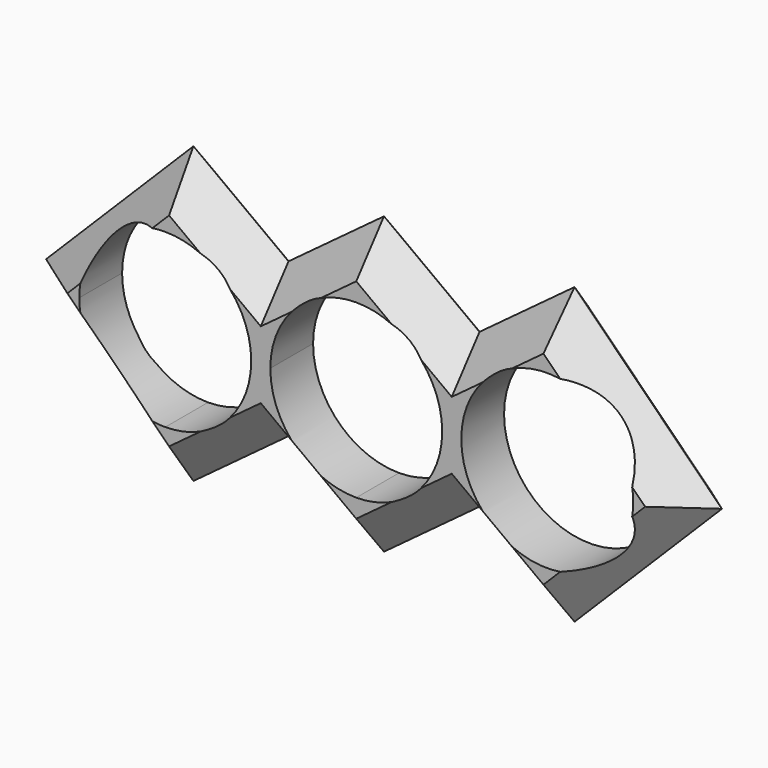
from build123d import *

# Parameters (mm, degrees)
F1_DEPTH      = 7
F2_T1_DEPTH   = 54.4125704052
F2_T3_DEPTH   = 54.4125704052
F2_T5_DEPTH   = 54.4125704052
F2_T7_DEPTH   = 54.4125704052
F2_T12_DEPTH  = 41.6814695772
F2_T17_DEPTH  = 41.6814695772
F2_T22_DEPTH  = 41.6814695772
F2_T27_DEPTH  = 41.6814695772
F2_T32_DEPTH  = 41.6814695772
F2_T37_DEPTH  = 41.6814695772
F2_T42_DEPTH  = 41.6814695772
F2_T47_DEPTH  = 41.6814695772
F2_T53_DEPTH  = 41.6814695772
F2_S55_R      = 11.25
F2_T56_DEPTH  = 25
F2_T59_DEPTH  = 41.6814695772
F2_S61_R      = 11.25
F2_T62_DEPTH  = 25
F2_T68_DEPTH  = 41.6814695772
F2_S70_R      = 11.25
F2_T71_DEPTH  = 25
F2_T74_DEPTH  = 41.6814695772
F2_S76_R      = 11.25
F2_T77_DEPTH  = 25
F2_T83_DEPTH  = 41.6814695772
F2_S85_R      = 11.25
F2_T86_DEPTH  = 25
F2_T89_DEPTH  = 41.6814695772
F2_S91_R      = 11.25
F2_T92_DEPTH  = 25
F2_T98_DEPTH  = 41.6814695772
F2_S100_R     = 11.25
F2_T101_DEPTH = 25
F2_T104_DEPTH = 41.6814695772
F2_S106_R     = 11.25
F2_T107_DEPTH = 25
F3_T1_DEPTH   = 43.7143691753
F3_T3_DEPTH   = 43.7143691753
F3_T5_DEPTH   = 43.7143691753
F3_T7_DEPTH   = 43.7143691753
F3_T12_DEPTH  = 30.9832683473
F3_T17_DEPTH  = 30.9832683473
F3_T22_DEPTH  = 30.9832683473
F3_T27_DEPTH  = 30.9832683473
F3_T32_DEPTH  = 30.9832683473
F3_T37_DEPTH  = 30.9832683473
F3_T42_DEPTH  = 30.9832683473
F3_T47_DEPTH  = 30.9832683473
F3_T53_DEPTH  = 30.9832683473
F3_T57_DEPTH  = 30.9832683473
F3_T64_DEPTH  = 30.9832683473
F3_T68_DEPTH  = 30.9832683473
F3_T75_DEPTH  = 30.9832683473
F3_T79_DEPTH  = 30.9832683473
F3_T86_DEPTH  = 30.9832683473
F3_T90_DEPTH  = 30.9832683473


# Not quite as in the source:
# - a fillet or chamfer that OpenCascade refuses, or shapes differently, is made with other operations: its cross-section is extruded or revolved along the edge and cut away or added


with BuildPart() as f1:
    # F0 (on Front) → F1 (new body)
    with BuildSketch(Plane.XZ):
        with BuildLine():
            Line((-25, 11.25), (-25, 20))
            Line((-25, 20), (-45, 0))
            Line((-45, 0), (-36.25, 0))
            ThreePointArc((-36.25, 0), (-32.9549512883, 7.9549512883), (-25, 11.25))
        make_face()
        with BuildLine():
            Line((-13.75, 0), (-12.5, 0))
            Line((-12.5, 0), (-12.5, 10.7452115044))
            Line((-12.5, 10.7452115044), (-25, 20))
            Line((-25, 20), (-25, 11.25))
            ThreePointArc((-25, 11.25), (-17.0450487117, 7.9549512883), (-13.75, 0))
        make_face()
        with BuildLine():
            Line((-12.5, -10.7452115044), (-12.5, 0))
            Line((-12.5, 0), (-13.75, 0))
            ThreePointArc((-13.75, 0), (-17.0450487117, -7.9549512883), (-25, -11.25))
            Line((-25, -11.25), (-25, -20))
            Line((-25, -20), (-12.5, -10.7452115044))
        make_face()
        with BuildLine():
            Line((-45, 0), (-25, -20))
            Line((-25, -20), (-25, -11.25))
            ThreePointArc((-25, -11.25), (-32.9549512883, -7.9549512883), (-36.25, 0))
            Line((-36.25, 0), (-45, 0))
        make_face()
        with BuildLine():
            Line((0, -20), (0, -11.25))
            ThreePointArc((0, -11.25), (-7.9549512883, -7.9549512883), (-11.25, 0))
            Line((-11.25, 0), (-12.5, 0))
            Line((-12.5, 0), (-12.5, -10.7452115044))
            Line((-12.5, -10.7452115044), (0, -20))
        make_face()
        with BuildLine():
            Line((12.5, 0), (11.25, 0))
            ThreePointArc((11.25, 0), (7.9549512883, -7.9549512883), (0, -11.25))
            Line((0, -11.25), (0, -20))
            Line((0, -20), (12.5, -10.7452115044))
            Line((12.5, -10.7452115044), (12.5, 0))
        make_face()
        with BuildLine():
            ThreePointArc((0, 11.25), (7.9549512883, 7.9549512883), (11.25, 0))
            Line((11.25, 0), (12.5, 0))
            Line((12.5, 0), (12.5, 10.7452115044))
            Line((12.5, 10.7452115044), (0, 20))
            Line((0, 20), (0, 11.25))
        make_face()
        with BuildLine():
            ThreePointArc((-11.25, 0), (-7.9549512883, 7.9549512883), (0, 11.25))
            Line((0, 11.25), (0, 20))
            Line((0, 20), (-12.5, 10.7452115044))
            Line((-12.5, 10.7452115044), (-12.5, 0))
            Line((-12.5, 0), (-11.25, 0))
        make_face()
        with BuildLine():
            Line((12.5, 10.7452115044), (12.5, 0))
            Line((12.5, 0), (13.75, 0))
            ThreePointArc((13.75, 0), (25, 11.25), (36.25, 0))
            Line((36.25, 0), (45, 0))
            Line((45, 0), (25, 20))
            Line((25, 20), (12.5, 10.7452115044))
        make_face()
        with BuildLine():
            Line((13.75, 0), (12.5, 0))
            Line((12.5, 0), (12.5, -10.7452115044))
            Line((12.5, -10.7452115044), (25, -20))
            Line((25, -20), (45, 0))
            Line((45, 0), (36.25, 0))
            ThreePointArc((36.25, 0), (25, -11.25), (13.75, 0))
        make_face()
    extrude(amount=F1_DEPTH)

    # F2: chamfer of 5.08 on 12 edges, made by hand

    # F2_s2 → F2_t1 (cut)
    with BuildSketch(Plane(origin=(6.7377487577, 0, 6.7377487577), x_dir=(0, 1, 0), z_dir=(-0.7071067812, 0, -0.7071067812))):
        Polygon((-1.92, -31.8198051534), (-7, -26.7398051534), (-7, -31.8198051534), align=None)
    extrude(amount=F2_T1_DEPTH, mode=Mode.SUBTRACT)

    # F2_s4 → F2_t3 (cut)
    with BuildSketch(Plane(origin=(31.7377487577, 0, -31.7377487577), x_dir=(0, 1, 0), z_dir=(-0.7071067812, 0, 0.7071067812))):
        Polygon((-1.92, -31.8198051534), (-7, -26.7398051534), (-7, -31.8198051534), align=None)
    extrude(amount=F2_T3_DEPTH, mode=Mode.SUBTRACT)

    # F2_s6 → F2_t5 (cut)
    with BuildSketch(Plane(origin=(-6.7377487577, 0, -6.7377487577), x_dir=(0, 1, 0), z_dir=(0.7071067812, 0, 0.7071067812))):
        Polygon((-1.92, -31.8198051534), (-7, -26.7398051534), (-7, -31.8198051534), align=None)
    extrude(amount=F2_T5_DEPTH, mode=Mode.SUBTRACT)

    # F2_s8 → F2_t7 (cut)
    with BuildSketch(Plane(origin=(-31.7377487577, 0, 31.7377487577), x_dir=(0, 1, 0), z_dir=(0.7071067812, 0, -0.7071067812))):
        Polygon((-1.92, -31.8198051534), (-7, -26.7398051534), (-7, -31.8198051534), align=None)
    extrude(amount=F2_T7_DEPTH, mode=Mode.SUBTRACT)


with BuildPart() as f2_tool10:
    # F2_s11 → F2_t12 (new body)
    with BuildSketch(Plane(origin=(-2.7131807604, 0, 2.008793127), x_dir=(0, 1, 0), z_dir=(-0.8036946592, 0, 0.5950419269))):
        Polygon((-1.92, -1.1978450121), (-7, 3.8821549879), (-7, -1.1978450121), align=None)
    extrude(amount=F2_T12_DEPTH)

    split(bisect_by=Plane(origin=(-9.5646403729, 0, 12.918502105), x_dir=(0, 1, 0), z_dir=(-0.5950419269, 0, 0.8036946592)), keep=Keep.TOP)


with BuildPart() as f1_1:
    add(f1.part)

    # F2_t9: cut F2_tool10
    add(f2_tool10.part, mode=Mode.SUBTRACT)


with BuildPart() as f2_tool15:
    # F2_s16 → F2_t17 (new body)
    with BuildSketch(Plane(origin=(20.0642276166, 0, 14.8552146336), x_dir=(0, 1, 0), z_dir=(-0.8036946592, 0, -0.5950419269))):
        Polygon((-1.92, -16.0738931843), (-7, -10.9938931843), (-7, -16.0738931843), align=None)
    extrude(amount=F2_T17_DEPTH)

    split(bisect_by=Plane(origin=(0.7127680041, 0, 0.9627016388), x_dir=(0, 1, 0), z_dir=(0.5950419269, 0, 0.8036946592)), keep=Keep.TOP)


with BuildPart() as f1_2:
    add(f1_1.part)

    # F2_t14: cut F2_tool15
    add(f2_tool15.part, mode=Mode.SUBTRACT)


with BuildPart() as f2_tool20:
    # F2_s21 → F2_t22 (new body)
    with BuildSketch(Plane(origin=(13.4349468708, 0, -9.9470073391), x_dir=(0, 1, 0), z_dir=(-0.8036946592, 0, 0.5950419269))):
        Polygon((-1.92, -16.0738931843), (-7, -10.9938931843), (-7, -16.0738931843), align=None)
    extrude(amount=F2_T22_DEPTH)

    split(bisect_by=Plane(origin=(-0.7127680041, 0, 0.9627016388), x_dir=(0, 1, 0), z_dir=(-0.5950419269, 0, 0.8036946592)), keep=Keep.TOP)


with BuildPart() as f1_3:
    add(f1_2.part)

    # F2_t19: cut F2_tool20
    add(f2_tool20.part, mode=Mode.SUBTRACT)


with BuildPart() as f2_tool25:
    # F2_s26 → F2_t27 (new body)
    with BuildSketch(Plane(origin=(36.2123552478, 0, 26.8110150997), x_dir=(0, 1, 0), z_dir=(-0.8036946592, 0, -0.5950419269))):
        Polygon((-1.92, -1.1978450121), (-7, 3.8821549879), (-7, -1.1978450121), align=None)
    extrude(amount=F2_T27_DEPTH)

    split(bisect_by=Plane(origin=(9.5646403729, 0, 12.918502105), x_dir=(0, 1, 0), z_dir=(0.5950419269, 0, 0.8036946592)), keep=Keep.TOP)


with BuildPart() as f1_4:
    add(f1_3.part)

    # F2_t24: cut F2_tool25
    add(f2_tool25.part, mode=Mode.SUBTRACT)


with BuildPart() as f2_tool30:
    # F2_s31 → F2_t32 (new body)
    with BuildSketch(Plane(origin=(2.7131807604, 0, -2.008793127), x_dir=(0, 1, 0), z_dir=(0.8036946592, 0, -0.5950419269))):
        Polygon((-1.92, -1.1978450121), (-7, 3.8821549879), (-7, -1.1978450121), align=None)
    extrude(amount=F2_T32_DEPTH)

    split(bisect_by=Plane(origin=(9.5646403729, 0, -12.918502105), x_dir=(0, 1, 0), z_dir=(0.5950419269, 0, -0.8036946592)), keep=Keep.TOP)


with BuildPart() as f1_5:
    add(f1_4.part)

    # F2_t29: cut F2_tool30
    add(f2_tool30.part, mode=Mode.SUBTRACT)


with BuildPart() as f2_tool35:
    # F2_s36 → F2_t37 (new body)
    with BuildSketch(Plane(origin=(-20.0642276166, 0, -14.8552146336), x_dir=(0, 1, 0), z_dir=(0.8036946592, 0, 0.5950419269))):
        Polygon((-1.92, -16.0738931843), (-7, -10.9938931843), (-7, -16.0738931843), align=None)
    extrude(amount=F2_T37_DEPTH)

    split(bisect_by=Plane(origin=(-0.7127680041, 0, -0.9627016388), x_dir=(0, 1, 0), z_dir=(-0.5950419269, 0, -0.8036946592)), keep=Keep.TOP)


with BuildPart() as f1_6:
    add(f1_5.part)

    # F2_t34: cut F2_tool35
    add(f2_tool35.part, mode=Mode.SUBTRACT)


with BuildPart() as f2_tool40:
    # F2_s41 → F2_t42 (new body)
    with BuildSketch(Plane(origin=(-13.4349468708, 0, 9.9470073391), x_dir=(0, 1, 0), z_dir=(0.8036946592, 0, -0.5950419269))):
        Polygon((-1.92, -16.0738931843), (-7, -10.9938931843), (-7, -16.0738931843), align=None)
    extrude(amount=F2_T42_DEPTH)

    split(bisect_by=Plane(origin=(0.7127680041, 0, -0.9627016388), x_dir=(0, 1, 0), z_dir=(0.5950419269, 0, -0.8036946592)), keep=Keep.TOP)


with BuildPart() as f1_7:
    add(f1_6.part)

    # F2_t39: cut F2_tool40
    add(f2_tool40.part, mode=Mode.SUBTRACT)


with BuildPart() as f2_tool45:
    # F2_s46 → F2_t47 (new body)
    with BuildSketch(Plane(origin=(-36.2123552478, 0, -26.8110150997), x_dir=(0, 1, 0), z_dir=(0.8036946592, 0, 0.5950419269))):
        Polygon((-1.92, -1.1978450121), (-7, 3.8821549879), (-7, -1.1978450121), align=None)
    extrude(amount=F2_T47_DEPTH)

    split(bisect_by=Plane(origin=(-9.5646403729, 0, -12.918502105), x_dir=(0, 1, 0), z_dir=(-0.5950419269, 0, -0.8036946592)), keep=Keep.TOP)


with BuildPart() as f1_8:
    add(f1_7.part)

    # F2_t44: cut F2_tool45
    add(f2_tool45.part, mode=Mode.SUBTRACT)


with BuildPart() as f2_tool51:
    # F2_s52 → F2_t53 (new body)
    with BuildSketch(Plane(origin=(20.0642276166, 0, 14.8552146336), x_dir=(0, 1, 0), z_dir=(-0.8036946592, 0, -0.5950419269))):
        Polygon((-1.92, -16.0738931843), (-7, -10.9938931843), (-7, -16.0738931843), align=None)
    extrude(amount=F2_T53_DEPTH)

    split(bisect_by=Plane(origin=(0.7127680041, 0, 0.9627016388), x_dir=(0, 1, 0), z_dir=(-0.5950419269, 0, -0.8036946592)), keep=Keep.TOP)

    # F2_s55 → F2_t56 (cut, symmetric)
    with BuildSketch(Plane.XZ.offset(4.5)):
        with Locations((-25, 0)):
            Circle(F2_S55_R)
    extrude(amount=F2_T56_DEPTH, both=True, mode=Mode.SUBTRACT)


with BuildPart() as f2_tool57:
    # F2_s58 → F2_t59 (new body)
    with BuildSketch(Plane(origin=(-2.7131807604, 0, 2.008793127), x_dir=(0, 1, 0), z_dir=(-0.8036946592, 0, 0.5950419269))):
        Polygon((-1.92, -1.1978450121), (-7, 3.8821549879), (-7, -1.1978450121), align=None)
    extrude(amount=F2_T59_DEPTH)

    split(bisect_by=Plane(origin=(-9.5646403729, 0, 12.918502105), x_dir=(0, 1, 0), z_dir=(0.5950419269, 0, -0.8036946592)), keep=Keep.TOP)

    # F2_s61 → F2_t62 (cut, symmetric)
    with BuildSketch(Plane.XZ.offset(4.5)):
        Circle(F2_S61_R)
    extrude(amount=F2_T62_DEPTH, both=True, mode=Mode.SUBTRACT)


with BuildPart() as f2_tool51_1:
    add(f2_tool51.part)

    # F2_t63: intersect F2_tool57
    add(f2_tool57.part, mode=Mode.INTERSECT)


with BuildPart() as f1_9:
    add(f1_8.part)

    # F2_t49: cut F2_tool51
    add(f2_tool51_1.part, mode=Mode.SUBTRACT)


with BuildPart() as f2_tool66:
    # F2_s67 → F2_t68 (new body)
    with BuildSketch(Plane(origin=(36.2123552478, 0, 26.8110150997), x_dir=(0, 1, 0), z_dir=(-0.8036946592, 0, -0.5950419269))):
        Polygon((-1.92, -1.1978450121), (-7, 3.8821549879), (-7, -1.1978450121), align=None)
    extrude(amount=F2_T68_DEPTH)

    split(bisect_by=Plane(origin=(9.5646403729, 0, 12.918502105), x_dir=(0, 1, 0), z_dir=(-0.5950419269, 0, -0.8036946592)), keep=Keep.TOP)

    # F2_s70 → F2_t71 (cut, symmetric)
    with BuildSketch(Plane.XZ.offset(4.5)):
        Circle(F2_S70_R)
    extrude(amount=F2_T71_DEPTH, both=True, mode=Mode.SUBTRACT)


with BuildPart() as f2_tool72:
    # F2_s73 → F2_t74 (new body)
    with BuildSketch(Plane(origin=(13.4349468708, 0, -9.9470073391), x_dir=(0, 1, 0), z_dir=(-0.8036946592, 0, 0.5950419269))):
        Polygon((-1.92, -16.0738931843), (-7, -10.9938931843), (-7, -16.0738931843), align=None)
    extrude(amount=F2_T74_DEPTH)

    split(bisect_by=Plane(origin=(-0.7127680041, 0, 0.9627016388), x_dir=(0, 1, 0), z_dir=(0.5950419269, 0, -0.8036946592)), keep=Keep.TOP)

    # F2_s76 → F2_t77 (cut, symmetric)
    with BuildSketch(Plane.XZ.offset(4.5)):
        with Locations((25, 0)):
            Circle(F2_S76_R)
    extrude(amount=F2_T77_DEPTH, both=True, mode=Mode.SUBTRACT)


with BuildPart() as f2_tool66_1:
    add(f2_tool66.part)

    # F2_t78: intersect F2_tool72
    add(f2_tool72.part, mode=Mode.INTERSECT)


with BuildPart() as f1_10:
    add(f1_9.part)

    # F2_t64: cut F2_tool66
    add(f2_tool66_1.part, mode=Mode.SUBTRACT)


with BuildPart() as f2_tool81:
    # F2_s82 → F2_t83 (new body)
    with BuildSketch(Plane(origin=(-20.0642276166, 0, -14.8552146336), x_dir=(0, 1, 0), z_dir=(0.8036946592, 0, 0.5950419269))):
        Polygon((-1.92, -16.0738931843), (-7, -10.9938931843), (-7, -16.0738931843), align=None)
    extrude(amount=F2_T83_DEPTH)

    split(bisect_by=Plane(origin=(-0.7127680041, 0, -0.9627016388), x_dir=(0, 1, 0), z_dir=(0.5950419269, 0, 0.8036946592)), keep=Keep.TOP)

    # F2_s85 → F2_t86 (cut, symmetric)
    with BuildSketch(Plane.XZ.offset(4.5)):
        with Locations((25, 0)):
            Circle(F2_S85_R)
    extrude(amount=F2_T86_DEPTH, both=True, mode=Mode.SUBTRACT)


with BuildPart() as f2_tool87:
    # F2_s88 → F2_t89 (new body)
    with BuildSketch(Plane(origin=(2.7131807604, 0, -2.008793127), x_dir=(0, 1, 0), z_dir=(0.8036946592, 0, -0.5950419269))):
        Polygon((-1.92, -1.1978450121), (-7, 3.8821549879), (-7, -1.1978450121), align=None)
    extrude(amount=F2_T89_DEPTH)

    split(bisect_by=Plane(origin=(9.5646403729, 0, -12.918502105), x_dir=(0, 1, 0), z_dir=(-0.5950419269, 0, 0.8036946592)), keep=Keep.TOP)

    # F2_s91 → F2_t92 (cut, symmetric)
    with BuildSketch(Plane.XZ.offset(4.5)):
        Circle(F2_S91_R)
    extrude(amount=F2_T92_DEPTH, both=True, mode=Mode.SUBTRACT)


with BuildPart() as f2_tool81_1:
    add(f2_tool81.part)

    # F2_t93: intersect F2_tool87
    add(f2_tool87.part, mode=Mode.INTERSECT)


with BuildPart() as f1_11:
    add(f1_10.part)

    # F2_t79: cut F2_tool81
    add(f2_tool81_1.part, mode=Mode.SUBTRACT)


with BuildPart() as f2_tool96:
    # F2_s97 → F2_t98 (new body)
    with BuildSketch(Plane(origin=(-36.2123552478, 0, -26.8110150997), x_dir=(0, 1, 0), z_dir=(0.8036946592, 0, 0.5950419269))):
        Polygon((-1.92, -1.1978450121), (-7, 3.8821549879), (-7, -1.1978450121), align=None)
    extrude(amount=F2_T98_DEPTH)

    split(bisect_by=Plane(origin=(-9.5646403729, 0, -12.918502105), x_dir=(0, 1, 0), z_dir=(0.5950419269, 0, 0.8036946592)), keep=Keep.TOP)

    # F2_s100 → F2_t101 (cut, symmetric)
    with BuildSketch(Plane.XZ.offset(4.5)):
        Circle(F2_S100_R)
    extrude(amount=F2_T101_DEPTH, both=True, mode=Mode.SUBTRACT)


with BuildPart() as f2_tool102:
    # F2_s103 → F2_t104 (new body)
    with BuildSketch(Plane(origin=(-13.4349468708, 0, 9.9470073391), x_dir=(0, 1, 0), z_dir=(0.8036946592, 0, -0.5950419269))):
        Polygon((-1.92, -16.0738931843), (-7, -10.9938931843), (-7, -16.0738931843), align=None)
    extrude(amount=F2_T104_DEPTH)

    split(bisect_by=Plane(origin=(0.7127680041, 0, -0.9627016388), x_dir=(0, 1, 0), z_dir=(-0.5950419269, 0, 0.8036946592)), keep=Keep.TOP)

    # F2_s106 → F2_t107 (cut, symmetric)
    with BuildSketch(Plane.XZ.offset(4.5)):
        with Locations((-25, 0)):
            Circle(F2_S106_R)
    extrude(amount=F2_T107_DEPTH, both=True, mode=Mode.SUBTRACT)


with BuildPart() as f2_tool96_1:
    add(f2_tool96.part)

    # F2_t108: intersect F2_tool102
    add(f2_tool102.part, mode=Mode.INTERSECT)


with BuildPart() as f1_12:
    add(f1_11.part)

    # F2_t94: cut F2_tool96
    add(f2_tool96_1.part, mode=Mode.SUBTRACT)

    # F3: chamfer of 3 on 12 edges, made by hand

    # F3_s2 → F3_t1 (cut)
    with BuildSketch(Plane(origin=(-2.9553634396, 0, -2.9553634396), x_dir=(0, 1, 0), z_dir=(0.7071067812, 0, 0.7071067812))):
        Polygon((0, -28.8198051534), (-3, -31.8198051534), (0, -31.8198051534), align=None)
    extrude(amount=F3_T1_DEPTH, mode=Mode.SUBTRACT)

    # F3_s4 → F3_t3 (cut)
    with BuildSketch(Plane(origin=(-27.9553634396, 0, 27.9553634396), x_dir=(0, 1, 0), z_dir=(0.7071067812, 0, -0.7071067812))):
        Polygon((0, -28.8198051534), (-3, -31.8198051534), (0, -31.8198051534), align=None)
    extrude(amount=F3_T3_DEPTH, mode=Mode.SUBTRACT)

    # F3_s6 → F3_t5 (cut)
    with BuildSketch(Plane(origin=(2.9553634396, 0, 2.9553634396), x_dir=(0, 1, 0), z_dir=(-0.7071067812, 0, -0.7071067812))):
        Polygon((-3, -31.8198051534), (0, -28.8198051534), (0, -31.8198051534), align=None)
    extrude(amount=F3_T5_DEPTH, mode=Mode.SUBTRACT)

    # F3_s8 → F3_t7 (cut)
    with BuildSketch(Plane(origin=(27.9553634396, 0, -27.9553634396), x_dir=(0, 1, 0), z_dir=(-0.7071067812, 0, 0.7071067812))):
        Polygon((0, -28.8198051534), (-3, -31.8198051534), (0, -31.8198051534), align=None)
    extrude(amount=F3_T7_DEPTH, mode=Mode.SUBTRACT)


with BuildPart() as f3_tool10:
    # F3_s11 → F3_t12 (new body)
    with BuildSketch(Plane(origin=(7.0122243563, 0, -5.1917322641), x_dir=(0, 1, 0), z_dir=(0.8036946592, 0, -0.5950419269))):
        Polygon((0, 1.8021549879), (-3, -1.1978450121), (0, -1.1978450121), align=None)
    extrude(amount=F3_T12_DEPTH)

    split(bisect_by=Plane(origin=(9.5646403729, 0, -12.918502105), x_dir=(0, 1, 0), z_dir=(0.5950419269, 0, -0.8036946592)), keep=Keep.TOP)


with BuildPart() as f1_13:
    add(f1_12.part)

    # F3_t9: cut F3_tool10
    add(f3_tool10.part, mode=Mode.SUBTRACT)


with BuildPart() as f3_tool15:
    # F3_s16 → F3_t17 (new body)
    with BuildSketch(Plane(origin=(-15.7651840208, 0, -11.6722754965), x_dir=(0, 1, 0), z_dir=(0.8036946592, 0, 0.5950419269))):
        Polygon((0, -13.0738931843), (-3, -16.0738931843), (0, -16.0738931843), align=None)
    extrude(amount=F3_T17_DEPTH)

    split(bisect_by=Plane(origin=(-0.7127680041, 0, -0.9627016388), x_dir=(0, 1, 0), z_dir=(-0.5950419269, 0, -0.8036946592)), keep=Keep.TOP)


with BuildPart() as f1_14:
    add(f1_13.part)

    # F3_t14: cut F3_tool15
    add(f3_tool15.part, mode=Mode.SUBTRACT)


with BuildPart() as f3_tool20:
    # F3_s21 → F3_t22 (new body)
    with BuildSketch(Plane(origin=(-9.1359032749, 0, 6.7640682021), x_dir=(0, 1, 0), z_dir=(0.8036946592, 0, -0.5950419269))):
        Polygon((0, -13.0738931843), (-3, -16.0738931843), (0, -16.0738931843), align=None)
    extrude(amount=F3_T22_DEPTH)

    split(bisect_by=Plane(origin=(0.7127680041, 0, -0.9627016388), x_dir=(0, 1, 0), z_dir=(0.5950419269, 0, -0.8036946592)), keep=Keep.TOP)


with BuildPart() as f1_15:
    add(f1_14.part)

    # F3_t19: cut F3_tool20
    add(f3_tool20.part, mode=Mode.SUBTRACT)


with BuildPart() as f3_tool25:
    # F3_s26 → F3_t27 (new body)
    with BuildSketch(Plane(origin=(-31.913311652, 0, -23.6280759627), x_dir=(0, 1, 0), z_dir=(0.8036946592, 0, 0.5950419269))):
        Polygon((0, 1.8021549879), (-3, -1.1978450121), (0, -1.1978450121), align=None)
    extrude(amount=F3_T27_DEPTH)

    split(bisect_by=Plane(origin=(-9.5646403729, 0, -12.918502105), x_dir=(0, 1, 0), z_dir=(-0.5950419269, 0, -0.8036946592)), keep=Keep.TOP)


with BuildPart() as f1_16:
    add(f1_15.part)

    # F3_t24: cut F3_tool25
    add(f3_tool25.part, mode=Mode.SUBTRACT)


with BuildPart() as f3_tool30:
    # F3_s31 → F3_t32 (new body)
    with BuildSketch(Plane(origin=(-7.0122243563, 0, 5.1917322641), x_dir=(0, 1, 0), z_dir=(-0.8036946592, 0, 0.5950419269))):
        Polygon((0, 1.8021549879), (-3, -1.1978450121), (0, -1.1978450121), align=None)
    extrude(amount=F3_T32_DEPTH)

    split(bisect_by=Plane(origin=(-9.5646403729, 0, 12.918502105), x_dir=(0, 1, 0), z_dir=(-0.5950419269, 0, 0.8036946592)), keep=Keep.TOP)


with BuildPart() as f1_17:
    add(f1_16.part)

    # F3_t29: cut F3_tool30
    add(f3_tool30.part, mode=Mode.SUBTRACT)


with BuildPart() as f3_tool35:
    # F3_s36 → F3_t37 (new body)
    with BuildSketch(Plane(origin=(15.7651840208, 0, 11.6722754965), x_dir=(0, 1, 0), z_dir=(-0.8036946592, 0, -0.5950419269))):
        Polygon((0, -13.0738931843), (-3, -16.0738931843), (0, -16.0738931843), align=None)
    extrude(amount=F3_T37_DEPTH)

    split(bisect_by=Plane(origin=(0.7127680041, 0, 0.9627016388), x_dir=(0, 1, 0), z_dir=(0.5950419269, 0, 0.8036946592)), keep=Keep.TOP)


with BuildPart() as f1_18:
    add(f1_17.part)

    # F3_t34: cut F3_tool35
    add(f3_tool35.part, mode=Mode.SUBTRACT)


with BuildPart() as f3_tool40:
    # F3_s41 → F3_t42 (new body)
    with BuildSketch(Plane(origin=(9.1359032749, 0, -6.7640682021), x_dir=(0, 1, 0), z_dir=(-0.8036946592, 0, 0.5950419269))):
        Polygon((0, -13.0738931843), (-3, -16.0738931843), (0, -16.0738931843), align=None)
    extrude(amount=F3_T42_DEPTH)

    split(bisect_by=Plane(origin=(-0.7127680041, 0, 0.9627016388), x_dir=(0, 1, 0), z_dir=(-0.5950419269, 0, 0.8036946592)), keep=Keep.TOP)


with BuildPart() as f1_19:
    add(f1_18.part)

    # F3_t39: cut F3_tool40
    add(f3_tool40.part, mode=Mode.SUBTRACT)


with BuildPart() as f3_tool45:
    # F3_s46 → F3_t47 (new body)
    with BuildSketch(Plane(origin=(31.913311652, 0, 23.6280759627), x_dir=(0, 1, 0), z_dir=(-0.8036946592, 0, -0.5950419269))):
        Polygon((0, 1.8021549879), (-3, -1.1978450121), (0, -1.1978450121), align=None)
    extrude(amount=F3_T47_DEPTH)

    split(bisect_by=Plane(origin=(9.5646403729, 0, 12.918502105), x_dir=(0, 1, 0), z_dir=(0.5950419269, 0, 0.8036946592)), keep=Keep.TOP)


with BuildPart() as f1_20:
    add(f1_19.part)

    # F3_t44: cut F3_tool45
    add(f3_tool45.part, mode=Mode.SUBTRACT)


with BuildPart() as f3_tool51:
    # F3_s52 → F3_t53 (new body)
    with BuildSketch(Plane(origin=(-15.7651840208, 0, -11.6722754965), x_dir=(0, 1, 0), z_dir=(0.8036946592, 0, 0.5950419269))):
        Polygon((0, -13.0738931843), (-3, -16.0738931843), (0, -16.0738931843), align=None)
    extrude(amount=F3_T53_DEPTH)

    split(bisect_by=Plane(origin=(-0.7127680041, 0, -0.9627016388), x_dir=(0, 1, 0), z_dir=(0.5950419269, 0, 0.8036946592)), keep=Keep.TOP)


with BuildPart() as f3_tool55:
    # F3_s56 → F3_t57 (new body)
    with BuildSketch(Plane(origin=(7.0122243563, 0, -5.1917322641), x_dir=(0, 1, 0), z_dir=(0.8036946592, 0, -0.5950419269))):
        Polygon((0, 1.8021549879), (-3, -1.1978450121), (0, -1.1978450121), align=None)
    extrude(amount=F3_T57_DEPTH)

    split(bisect_by=Plane(origin=(9.5646403729, 0, -12.918502105), x_dir=(0, 1, 0), z_dir=(-0.5950419269, 0, 0.8036946592)), keep=Keep.TOP)


with BuildPart() as f3_tool51_1:
    add(f3_tool51.part)

    # F3_t59: intersect F3_tool55
    add(f3_tool55.part, mode=Mode.INTERSECT)


with BuildPart() as f1_21:
    add(f1_20.part)

    # F3_t49: cut F3_tool51
    add(f3_tool51_1.part, mode=Mode.SUBTRACT)


with BuildPart() as f3_tool62:
    # F3_s63 → F3_t64 (new body)
    with BuildSketch(Plane(origin=(-31.913311652, 0, -23.6280759627), x_dir=(0, 1, 0), z_dir=(0.8036946592, 0, 0.5950419269))):
        Polygon((0, 1.8021549879), (-3, -1.1978450121), (0, -1.1978450121), align=None)
    extrude(amount=F3_T64_DEPTH)

    split(bisect_by=Plane(origin=(-9.5646403729, 0, -12.918502105), x_dir=(0, 1, 0), z_dir=(0.5950419269, 0, 0.8036946592)), keep=Keep.TOP)


with BuildPart() as f3_tool66:
    # F3_s67 → F3_t68 (new body)
    with BuildSketch(Plane(origin=(-9.1359032749, 0, 6.7640682021), x_dir=(0, 1, 0), z_dir=(0.8036946592, 0, -0.5950419269))):
        Polygon((0, -13.0738931843), (-3, -16.0738931843), (0, -16.0738931843), align=None)
    extrude(amount=F3_T68_DEPTH)

    split(bisect_by=Plane(origin=(0.7127680041, 0, -0.9627016388), x_dir=(0, 1, 0), z_dir=(-0.5950419269, 0, 0.8036946592)), keep=Keep.TOP)


with BuildPart() as f3_tool62_1:
    add(f3_tool62.part)

    # F3_t70: intersect F3_tool66
    add(f3_tool66.part, mode=Mode.INTERSECT)


with BuildPart() as f1_22:
    add(f1_21.part)

    # F3_t60: cut F3_tool62
    add(f3_tool62_1.part, mode=Mode.SUBTRACT)


with BuildPart() as f3_tool73:
    # F3_s74 → F3_t75 (new body)
    with BuildSketch(Plane(origin=(15.7651840208, 0, 11.6722754965), x_dir=(0, 1, 0), z_dir=(-0.8036946592, 0, -0.5950419269))):
        Polygon((0, -13.0738931843), (-3, -16.0738931843), (0, -16.0738931843), align=None)
    extrude(amount=F3_T75_DEPTH)

    split(bisect_by=Plane(origin=(0.7127680041, 0, 0.9627016388), x_dir=(0, 1, 0), z_dir=(-0.5950419269, 0, -0.8036946592)), keep=Keep.TOP)


with BuildPart() as f3_tool77:
    # F3_s78 → F3_t79 (new body)
    with BuildSketch(Plane(origin=(-7.0122243563, 0, 5.1917322641), x_dir=(0, 1, 0), z_dir=(-0.8036946592, 0, 0.5950419269))):
        Polygon((0, 1.8021549879), (-3, -1.1978450121), (0, -1.1978450121), align=None)
    extrude(amount=F3_T79_DEPTH)

    split(bisect_by=Plane(origin=(-9.5646403729, 0, 12.918502105), x_dir=(0, 1, 0), z_dir=(0.5950419269, 0, -0.8036946592)), keep=Keep.TOP)


with BuildPart() as f3_tool73_1:
    add(f3_tool73.part)

    # F3_t81: intersect F3_tool77
    add(f3_tool77.part, mode=Mode.INTERSECT)


with BuildPart() as f1_23:
    add(f1_22.part)

    # F3_t71: cut F3_tool73
    add(f3_tool73_1.part, mode=Mode.SUBTRACT)


with BuildPart() as f3_tool84:
    # F3_s85 → F3_t86 (new body)
    with BuildSketch(Plane(origin=(31.913311652, 0, 23.6280759627), x_dir=(0, 1, 0), z_dir=(-0.8036946592, 0, -0.5950419269))):
        Polygon((0, 1.8021549879), (-3, -1.1978450121), (0, -1.1978450121), align=None)
    extrude(amount=F3_T86_DEPTH)

    split(bisect_by=Plane(origin=(9.5646403729, 0, 12.918502105), x_dir=(0, 1, 0), z_dir=(-0.5950419269, 0, -0.8036946592)), keep=Keep.TOP)


with BuildPart() as f3_tool88:
    # F3_s89 → F3_t90 (new body)
    with BuildSketch(Plane(origin=(9.1359032749, 0, -6.7640682021), x_dir=(0, 1, 0), z_dir=(-0.8036946592, 0, 0.5950419269))):
        Polygon((0, -13.0738931843), (-3, -16.0738931843), (0, -16.0738931843), align=None)
    extrude(amount=F3_T90_DEPTH)

    split(bisect_by=Plane(origin=(-0.7127680041, 0, 0.9627016388), x_dir=(0, 1, 0), z_dir=(0.5950419269, 0, -0.8036946592)), keep=Keep.TOP)


with BuildPart() as f3_tool84_1:
    add(f3_tool84.part)

    # F3_t92: intersect F3_tool88
    add(f3_tool88.part, mode=Mode.INTERSECT)


with BuildPart() as f1_24:
    add(f1_23.part)

    # F3_t82: cut F3_tool84
    add(f3_tool84_1.part, mode=Mode.SUBTRACT)


solid = f1_24.part
